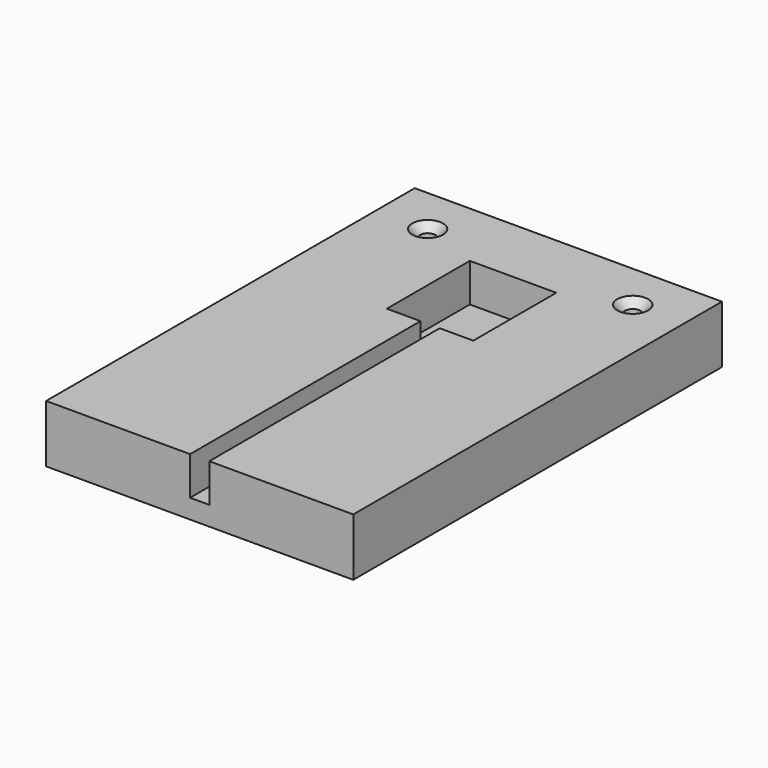
from build123d import *

# Parameters (mm, degrees)
F0_W           = 80
F0_H           = 120
F1_DEPTH       = 15
F3_DEPTH       = 10
F5_D           = 4
F5_CSINK_D     = 8
F5_CSINK_ANGLE = 90


with BuildPart() as f1:
    # F0 (on Top) → F1 (new body)
    with BuildSketch(Plane.XY):
        Rectangle(F0_W, F0_H)
    extrude(amount=F1_DEPTH)

    # F2 (on face) → F3 (cut)
    with BuildSketch(Plane.XY.offset(15)):
        Polygon((-11.2589411438, 15), (-2.5, 15), (-2.5, -60), (0, -60), (2.5, -60), (2.5, 15), (11.2589411438, 15), (11.2589411438, 42), (-11.2589411438, 42), align=None)
    extrude(amount=-F3_DEPTH, mode=Mode.SUBTRACT)

    # F5 (through all)
    with Locations(Plane.XY.offset(15)):
        with Locations((-26.7064720392, 47.5818291306), (26.7064720392, 47.5818291306)):
            CounterSinkHole(F5_D / 2, F5_CSINK_D / 2, counter_sink_angle=F5_CSINK_ANGLE)


solid = f1.part
